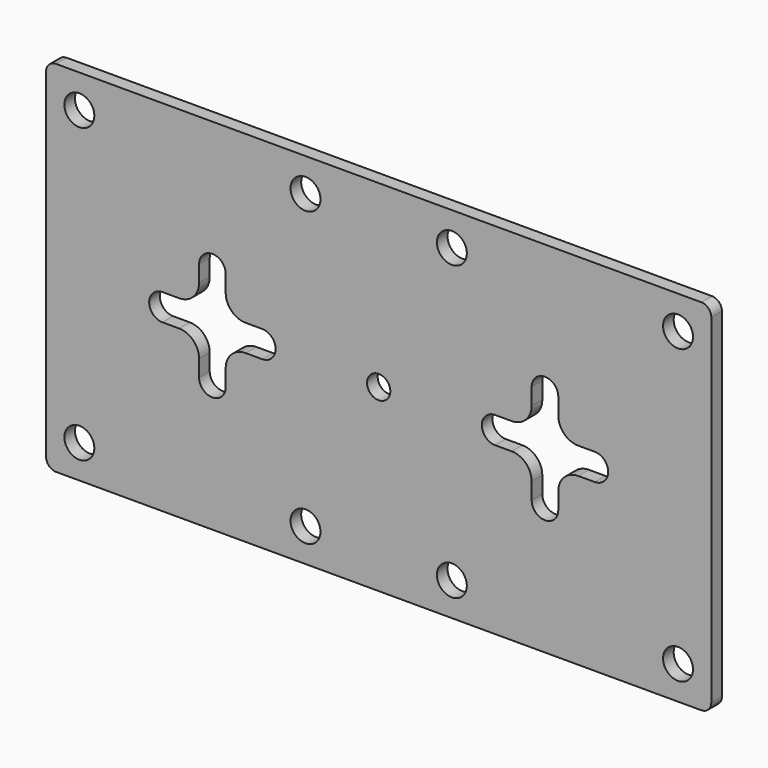
from build123d import *

# Parameters (mm, degrees)
F0_W     = 100
F0_H     = 54
F0_R     = 2.25
F1_DEPTH = 2
F2_W     = 2
F2_H     = 2
F2_R     = 1.75
F3_DEPTH = 2
F4_R     = 3
F5_R     = 1.5


# Not quite as in the source:
# - a feature names something its author has since deleted; it is built from what else it names


with BuildPart() as f1:
    # F0 (on Front) → F1 (new body)
    with BuildSketch(Plane.XZ):
        with Locations((50, 27)):
            Rectangle(F0_W, F0_H)
        with Locations((5, 5)):
            Circle(F0_R, mode=Mode.SUBTRACT)
        with Locations((39, 5)):
            Circle(F0_R, mode=Mode.SUBTRACT)
        with Locations((61, 5)):
            Circle(F0_R, mode=Mode.SUBTRACT)
        with Locations((95, 5)):
            Circle(F0_R, mode=Mode.SUBTRACT)
        with Locations((5, 49)):
            Circle(F0_R, mode=Mode.SUBTRACT)
        with Locations((39, 49)):
            Circle(F0_R, mode=Mode.SUBTRACT)
        with Locations((61, 49)):
            Circle(F0_R, mode=Mode.SUBTRACT)
        with Locations((95, 49)):
            Circle(F0_R, mode=Mode.SUBTRACT)
    extrude(amount=F1_DEPTH)

    # F2 (on face) → F3 (cut)
    with BuildSketch(Plane.XZ.offset(2)):
        with Locations((24, 28)):
            Rectangle(F2_W, F2_H)
        with BuildLine():
            Line((23, 25), (23, 27))
            Line((23, 27), (23, 29))
            Line((23, 29), (17.5, 29))
            ThreePointArc((17.5, 29), (15.5, 27), (17.5, 25))
            Line((17.5, 25), (23, 25))
        make_face()
        with Locations((24, 26)):
            Rectangle(F2_W, F2_H)
        with Locations((26, 28)):
            Rectangle(F2_W, F2_H)
        with Locations((26, 26)):
            Rectangle(F2_W, F2_H)
        with BuildLine():
            Line((23, 34.5), (23, 29))
            Line((23, 29), (25, 29))
            Line((25, 29), (27, 29))
            Line((27, 29), (27, 34.5))
            ThreePointArc((27, 34.5), (25, 36.5), (23, 34.5))
        make_face()
        with BuildLine():
            Line((25, 25), (23, 25))
            Line((23, 25), (23, 19.5))
            ThreePointArc((23, 19.5), (25, 17.5), (27, 19.5))
            Line((27, 19.5), (27, 25))
            Line((27, 25), (25, 25))
        make_face()
        with BuildLine():
            Line((27, 29), (27, 27))
            Line((27, 27), (27, 25))
            Line((27, 25), (32.5, 25))
            ThreePointArc((32.5, 25), (34.5, 27), (32.5, 29))
            Line((32.5, 29), (27, 29))
        make_face()
        with Locations((50, 27)):
            Circle(F2_R)
        with Locations((74, 28)):
            Rectangle(F2_W, F2_H)
        with BuildLine():
            Line((73, 25), (73, 27))
            Line((73, 27), (73, 29))
            Line((73, 29), (67.5, 29))
            ThreePointArc((67.5, 29), (65.5, 27), (67.5, 25))
            Line((67.5, 25), (73, 25))
        make_face()
        with Locations((74, 26)):
            Rectangle(F2_W, F2_H)
        with Locations((76, 28)):
            Rectangle(F2_W, F2_H)
        with Locations((76, 26)):
            Rectangle(F2_W, F2_H)
        with BuildLine():
            Line((73, 34.5), (73, 29))
            Line((73, 29), (75, 29))
            Line((75, 29), (77, 29))
            Line((77, 29), (77, 34.5))
            ThreePointArc((77, 34.5), (75, 36.5), (73, 34.5))
        make_face()
        with BuildLine():
            Line((75, 25), (73, 25))
            Line((73, 25), (73, 19.5))
            ThreePointArc((73, 19.5), (75, 17.5), (77, 19.5))
            Line((77, 19.5), (77, 25))
            Line((77, 25), (75, 25))
        make_face()
        with BuildLine():
            Line((77, 29), (77, 27))
            Line((77, 27), (77, 25))
            Line((77, 25), (82.5, 25))
            ThreePointArc((82.5, 25), (84.5, 27), (82.5, 29))
            Line((82.5, 29), (77, 29))
        make_face()
    extrude(amount=-F3_DEPTH, mode=Mode.SUBTRACT)

    # F4
    f4_edges = [f1.edges().sort_by_distance(p)[0] for p in [
        (23, -1, 29),
        (23, -1, 25),
        (27, -1, 25),
        (27, -1, 29),
        (73, -1, 29),
        (77, -1, 29),
        (77, -1, 25),
        (73, -1, 25),
    ]]
    fillet(f4_edges, radius=F4_R)

    # F5
    f5_edges = [f1.edges().sort_by_distance(p)[0] for p in [
        (0, -1, 54),
        (0, -1, 0),
        (100, -1, 54),
        (100, -1, 0),
    ]]
    fillet(f5_edges, radius=F5_R)


solid = f1.part
